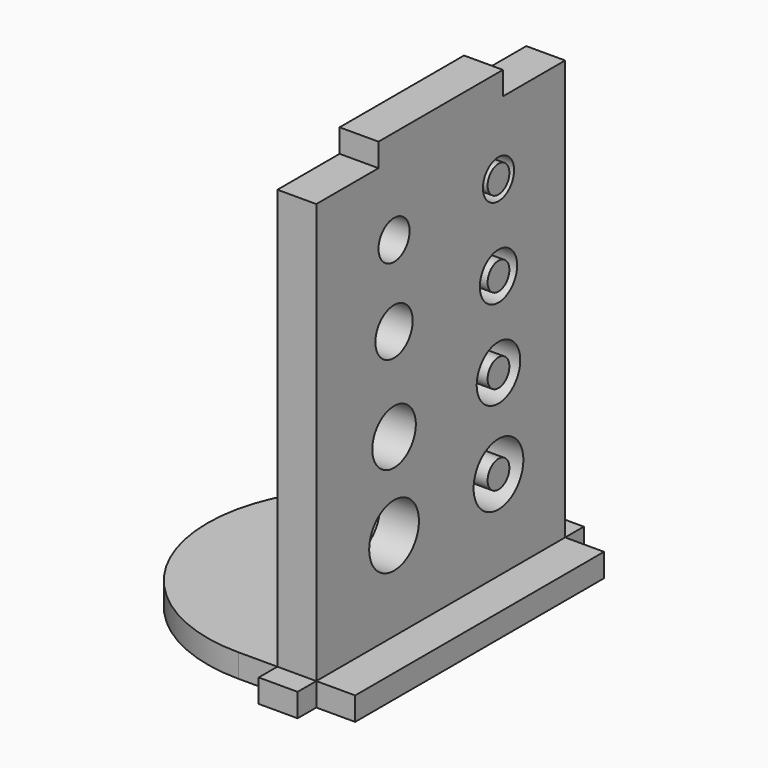
from build123d import *

# Parameters (mm, degrees)
F0_W     = 5
F0_H     = 3
F0_H_2   = 10
F1_DEPTH = 3
F0_H_3   = 20
F2_DEPTH = 60
F3_DEPTH = 3
F4_W     = 5
F4_H     = 10
F5_DEPTH = 3
F6_R     = 2.5
F6_R_2   = 3
F6_R_3   = 3.5
F6_R_4   = 4
F6_R_5   = 1.75
F7_DEPTH = 5


with BuildPart() as f1:
    # F0 (on Top) → F1 (new body)
    with BuildSketch(Plane.XY):
        with BuildLine():
            Line((-7.5, -20), (-7.5, 20))
            ThreePointArc((-7.5, 20), (-27.5, 0), (-7.5, -20))
        make_face()
        Polygon((7.5, -20), (7.5, 20), (2.5, 20), (2.5, 10), (2.5, -10), (2.5, -20), align=None)
        with Locations((0, 21.5)):
            Rectangle(F0_W, F0_H)
        with Locations((0, -21.5)):
            Rectangle(F0_W, F0_H)
        Polygon((-2.5, 10), (-2.5, 20), (-7.5, 20), (-7.5, -20), (-2.5, -20), (-2.5, -10), align=None)
        with Locations((0, 15)):
            Rectangle(F0_W, F0_H_2)
        with Locations((0, -15)):
            Rectangle(F0_W, F0_H_2)
    extrude(amount=F1_DEPTH)


with BuildPart() as f2:
    # F0 (on Top) → F2 (new body)
    with BuildSketch(Plane.XY):
        Rectangle(F0_W, F0_H_3)
        with Locations((0, 15)):
            Rectangle(F0_W, F0_H_2)
        with Locations((0, -15)):
            Rectangle(F0_W, F0_H_2)
    extrude(amount=F2_DEPTH)

    # F0 (on Top) → F3 (cut)
    with BuildSketch(Plane.XY):
        with Locations((0, 15)):
            Rectangle(F0_W, F0_H_2)
        with Locations((0, -15)):
            Rectangle(F0_W, F0_H_2)
    extrude(amount=F3_DEPTH, mode=Mode.SUBTRACT)

    # F4 (on face) → F5 (cut)
    with BuildSketch(Plane.XY.offset(60)):
        with Locations((0, -15)):
            Rectangle(F4_W, F4_H)
        with Locations((0, 15)):
            Rectangle(F4_W, F4_H)
    extrude(amount=-F5_DEPTH, mode=Mode.SUBTRACT)

    # F6 (on face) → F7 (cut, through all)
    with BuildSketch(Plane(origin=(-2.5, 0, 0), x_dir=(0, -1, 0), z_dir=(-1, 0, 0))):
        with Locations((7.5, 47.8578992188)):
            Circle(F6_R)
        with Locations((7.5, 37.4925732613)):
            Circle(F6_R_2)
        with Locations((7.5, 25.5654416978)):
            Circle(F6_R_3)
        with Locations((7.5, 14.4113665447)):
            Circle(F6_R_4)
        with Locations((-9.2865563929, 14.5218027756)):
            Circle(F6_R_4)
        with Locations((-9.2865563929, 14.5218027756)):
            Circle(F6_R_5, mode=Mode.SUBTRACT)
        with Locations((-9.2865563929, 26.0071866214)):
            Circle(F6_R_3)
        with Locations((-9.2865563929, 26.0071866214)):
            Circle(F6_R_5, mode=Mode.SUBTRACT)
        with Locations((-9.2865563929, 36.9403921068)):
            Circle(F6_R_2)
        with Locations((-9.2865563929, 36.9403921068)):
            Circle(F6_R_5, mode=Mode.SUBTRACT)
        with Locations((-9.2865563929, 47.9186363518)):
            Circle(F6_R)
        with Locations((-9.2865563929, 47.9186363518)):
            Circle(F6_R_5, mode=Mode.SUBTRACT)
    extrude(amount=-F7_DEPTH, mode=Mode.SUBTRACT)


solid = Compound([f1.part, f2.part])
